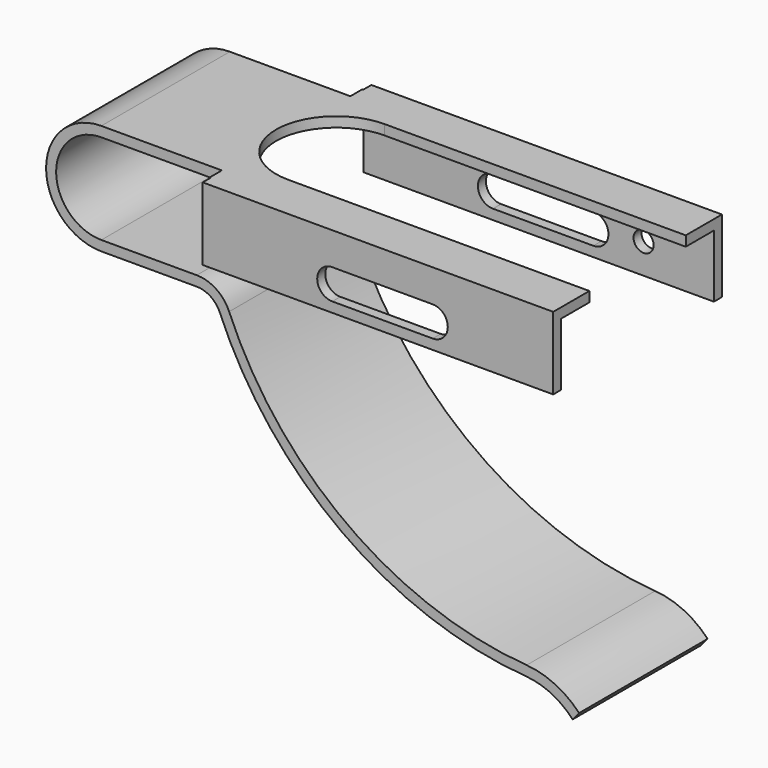
from build123d import *

# Parameters (mm, degrees)
F1_DEPTH  = 16
F3_W      = 70
F3_H      = 3
F4_DEPTH  = 2
F5_W      = 69.8145667315
F5_H      = 14.4820966907
F6_DEPTH  = 2
F9_DEPTH  = 2
F11_DEPTH = 42.001
F13_D     = 4
F13_DEPTH = 21.001
F14_R     = 3
F14_R_2   = 2
F15_DEPTH = 5


with BuildPart() as f1:
    # F0 (on Front) → F1 (new body)
    with BuildSketch(Plane.XZ):
        with BuildLine():
            Line((94, 11), (0, 11))
            ThreePointArc((0, 11), (-11, 0), (0, -11))
            Line((0, -11), (19, -11))
            ThreePointArc((19, -11), (21.7681124643, -11.8361612201), (23.6103896104, -14.064978646))
            ThreePointArc((23.6103896104, -14.064978646), (47.8977113224, -44.6078392712), (84.5520957277, -57.9942665386))
            ThreePointArc((84.5520957277, -57.9942665386), (89.6419160729, -59.3768457194), (93.8590048523, -62.5444881493))
            Line((93.8590048523, -62.5444881493), (95.1549842887, -61))
            ThreePointArc((95.1549842887, -61), (90.3976747979, -57.5207528796), (84.7034264019, -56))
            ThreePointArc((84.7034264019, -56), (49.0672193413, -42.9854179344), (25.4545454545, -13.2909701044))
            ThreePointArc((25.4545454545, -13.2909701044), (22.87535745, -10.1706257081), (19, -9))
            Line((19, -9), (0, -9))
            ThreePointArc((0, -9), (-9, 0), (0, 9))
            Line((0, 9), (94, 9))
            Line((94, 9), (94, 11))
        make_face()
    extrude(amount=F1_DEPTH)

    # F3 (on face) → F4 (join)
    with BuildSketch(Plane.XY.offset(11)):
        with Locations((59, -17.5)):
            Rectangle(F3_W, F3_H)
    extrude(amount=-F4_DEPTH)

    # F5 (on face) → F6 (join)
    with BuildSketch(Plane.XZ.offset(19)):
        with Locations((59.0927166343, 3.7589516547)):
            Rectangle(F5_W, F5_H)
    extrude(amount=F6_DEPTH)

    # F7: F1 across face


with BuildPart() as f1_1:
    add(f1.part)
    add(f1.part.mirror(Plane.XZ))

    # F8 (on face) → F9 (cut)
    with BuildSketch(Plane.XY.offset(11)):
        with BuildLine():
            Line((94, 12), (34, 12))
            ThreePointArc((34, 12), (22, 0), (34, -12))
            Line((34, -12), (94, -12))
            Line((94, -12), (94, 12))
        make_face()
    extrude(amount=-F9_DEPTH, mode=Mode.SUBTRACT)

    # F10 (on face) → F11 (cut, through all)
    with BuildSketch(Plane.XZ.offset(21)):
        with BuildLine():
            ThreePointArc((50, 4.5179033093), (47, 1.5179033093), (50, -1.4820966907))
            Line((50, -1.4820966907), (70, -1.4820966907))
            ThreePointArc((70, -1.4820966907), (73, 1.5179033093), (70, 4.5179033093))
            Line((70, 4.5179033093), (50, 4.5179033093))
        make_face()
    extrude(amount=-F11_DEPTH, mode=Mode.SUBTRACT)

    # F13 (through all, one way)
    with BuildSketch(Plane.XZ):
        with Locations((80, 2.5179033093)):
            Circle(F13_D / 2)
    extrude(amount=-F13_DEPTH, mode=Mode.SUBTRACT)

    # F14 (on face) → F15 (join)
    with BuildSketch(Plane(origin=(0, -19, 0), x_dir=(-1, 0, 0), z_dir=(0, 1, 0))):
        with Locations((-80, 2.5179033093)):
            Circle(F14_R)
        with Locations((-80, 2.5179033093)):
            Circle(F14_R_2, mode=Mode.SUBTRACT)
    extrude(amount=F15_DEPTH)


solid = f1_1.part
